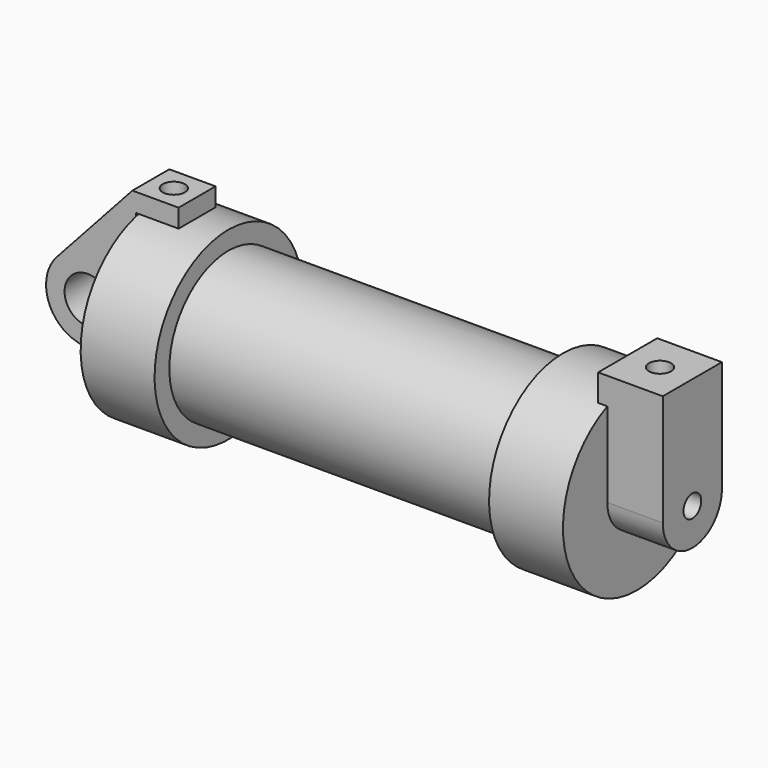
from build123d import *

# Parameters (mm, degrees)
F0_W      = 5.842
F0_H      = 12.7
F0_R      = 3.175
F3_DEPTH  = 3.175
F4_R      = 1.524
F5_DEPTH  = 7.62
F6_DEPTH  = 1.27
F8_R      = 1.524
F9_DEPTH  = 10.414
F10_DEPTH = 11.9279641658
F7_R      = 1.524
F11_DEPTH = 9.9806375802


with BuildPart() as f2:
    # F0 (on Front) → F2 (revolve)
    with BuildSketch(Plane.XZ):
        Polygon((5.842, 12.7), (5.842, 0), (66.294, 0), (66.294, 12.7), (56.134, 12.7), (56.134, 10.16), (10.16, 10.16), (10.16, 12.7), align=None)
        with Locations((2.921, 6.35)):
            Rectangle(F0_W, F0_H)
    revolve(axis=Axis((33.147, 0, 0), (-1, 0, 0)))

    # F4 (on face) → F5 (join)
    with BuildSketch(Plane.YZ.offset(66.294)):
        with BuildLine():
            ThreePointArc((-5.08, 0), (0, -5.08), (5.08, 0))
            ThreePointArc((5.08, 0), (0, 5.08), (-5.08, 0))
        make_face()
        Circle(F4_R, mode=Mode.SUBTRACT)
        with BuildLine():
            ThreePointArc((-5.08, 0), (0, 5.08), (5.08, 0))
            Line((5.08, 0), (5.08, 15.3334243223))
            Line((5.08, 15.3334243223), (-5.08, 15.3334243223))
            Line((-5.08, 15.3334243223), (-5.08, 0))
        make_face()
    extrude(amount=F5_DEPTH)

    # F6 (add): a face of the model
    f6_faces = [f2.faces().sort_by_distance(p)[0] for p in [
        (66.294, 0, 13.8265158547),
    ]]
    extrude(f6_faces, amount=F6_DEPTH)

    # F8 (on face) → F9 (join)
    with BuildSketch(Plane.XY.offset(15.3334243223)):
        with Locations((69.469, 0)):
            Circle(F8_R)
    extrude(amount=-F9_DEPTH)

    # F8 (on face) → F10 (cut)
    with BuildSketch(Plane.XY.offset(15.3334243223)):
        with Locations((69.469, 0)):
            Circle(F8_R)
    extrude(amount=-F10_DEPTH, mode=Mode.SUBTRACT)


with BuildPart() as f3:
    # F0 (on Front) → F3 (new body, symmetric)
    with BuildSketch(Plane.XZ):
        with BuildLine():
            Line((-0.9398, 0), (0, 0))
            Line((0, 0), (0, 12.7))
            Line((0, 12.7), (5.842, 12.7))
            Line((5.842, 12.7), (5.842, 15.24))
            Line((5.842, 15.24), (-0.508, 15.24))
            Line((-0.508, 15.24), (-10.8806298187, 3.8475430269))
            ThreePointArc((-10.8806298187, 3.8475430269), (-4.5919612295, 5.3297205562), (-0.9398, 0))
        make_face()
        with BuildLine():
            Line((5.842, 0), (0, 0))
            Line((0, 0), (-0.9398, 0))
            ThreePointArc((-0.9398, 0), (-3.1957909266, -4.5493385486), (-8.1826630726, -5.5069827884))
            Line((-8.1826630726, -5.5069827884), (5.842, -9.398))
            Line((5.842, -9.398), (5.842, 0))
        make_face()
        with BuildLine():
            ThreePointArc((-8.1826630726, -5.5069827884), (-3.1957909266, -4.5493385486), (-0.9398, 0))
            ThreePointArc((-0.9398, 0), (-4.5919612295, 5.3297205562), (-10.8806298187, 3.8475430269))
            ThreePointArc((-10.8806298187, 3.8475430269), (-12.1459778134, -1.5837270034), (-8.1826630726, -5.5069827884))
        make_face()
        with Locations((-6.6548, 0)):
            Circle(F0_R, mode=Mode.SUBTRACT)
    extrude(amount=F3_DEPTH, both=True)

    # F7 (on face) → F11 (cut)
    with BuildSketch(Plane.XY.offset(15.24)):
        with Locations((2.6162154973, 0.0347092391)):
            Circle(F7_R)
    extrude(amount=-F11_DEPTH, mode=Mode.SUBTRACT)


solid = Compound([f2.part, f3.part])
